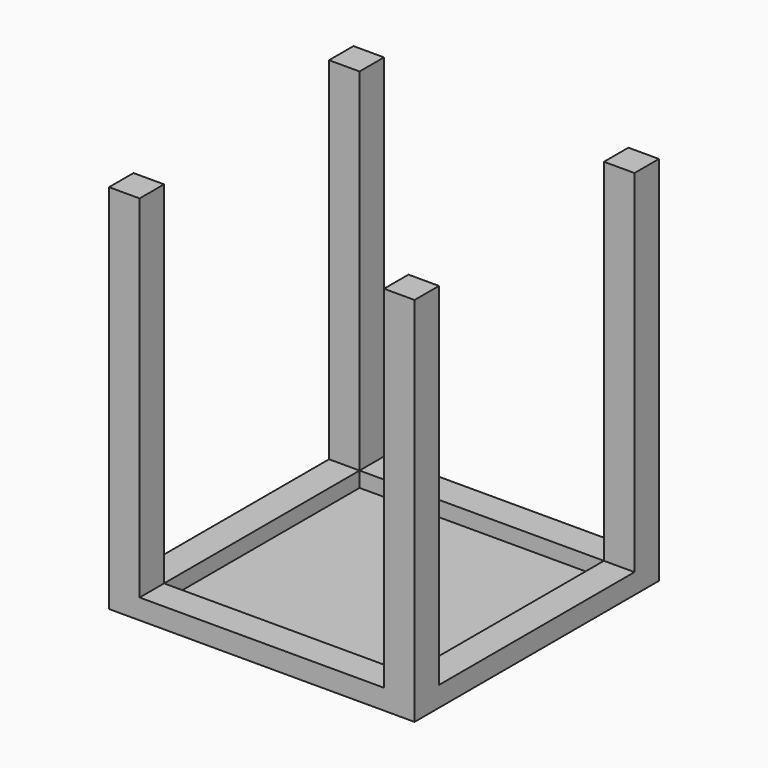
from build123d import *

# Parameters (mm, degrees)
F0_W     = 400
F0_H     = 400
F1_DEPTH = 6.35
F2_W     = 400
F2_H     = 400
F2_W_2   = 320
F2_H_2   = 320
F3_DEPTH = 20
F4_W     = 40
F4_H     = 40
F5_DEPTH = 460


# Not quite as in the source:
# - a length typed as a fraction of an inch, garbled in the dataset ("3 / 203.2 mm" for 3/8 in), is restored


with BuildPart() as f1:
    # F0 (on Top) → F1 (new body)
    with BuildSketch(Plane.XY):
        with Locations((200, 200)):
            Rectangle(F0_W, F0_H)
    extrude(amount=F1_DEPTH)

    # F2 (on face) → F3 (join)
    with BuildSketch(Plane.XY.offset(6.35)):
        with Locations((200, 200)):
            Rectangle(F2_W, F2_H)
        with Locations((200, 200)):
            Rectangle(F2_W_2, F2_H_2, mode=Mode.SUBTRACT)
    extrude(amount=F3_DEPTH)

    # F4 (on face) → F5 (join)
    with BuildSketch(Plane.XY.offset(26.35)):
        with Locations((20, 380)):
            Rectangle(F4_W, F4_H)
        with Locations((380, 380)):
            Rectangle(F4_W, F4_H)
        with Locations((380, 20)):
            Rectangle(F4_W, F4_H)
        with Locations((20, 20)):
            Rectangle(F4_W, F4_H)
    extrude(amount=F5_DEPTH)


solid = f1.part
